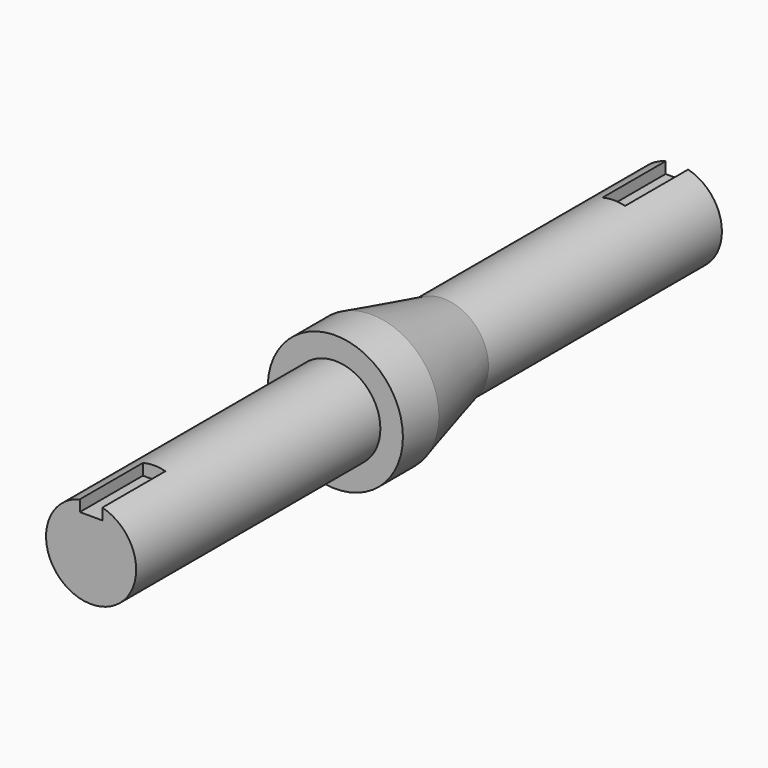
from build123d import *

# Parameters (mm, degrees)
F0_R     = 4
F1_DEPTH = 65
F3_R     = 6
F4_DEPTH = 4
F5_SIZE2 = 1.99999
F5_SIZE  = 7.99999
F7_DEPTH = 7


# Not quite as in the source:
# - a fillet or chamfer is up to 0.001 mm smaller than in the source, because OpenCascade refuses the exact size
# - a pattern or mirror of a feature is missing from the dataset's text; its kind, count and spacing are read off the source's solid


with BuildPart() as f1:
    # F0 (on Front) → F1 (new body)
    with BuildSketch(Plane.XZ):
        Circle(F0_R)
    extrude(amount=F1_DEPTH)

    # F3 (on offset) → F4 (join)
    with BuildSketch(Plane.XZ.offset(37.9)):
        Circle(F3_R)
    extrude(amount=-F4_DEPTH)

    # F5 (size 8 and 2 in the source; OpenCascade refuses exactly that, so slightly less here)
    f5_edges = [f1.edges().sort_by_distance(p)[0] for p in [
        (-4, -33.9, 0),
    ]]
    f5_side = f1.faces().sort_by_distance((-4, -16.95, 0))[0]
    chamfer(f5_edges, length=F5_SIZE, length2=F5_SIZE2, reference=f5_side)

    # F6 (on face) → F7 (cut)
    with BuildSketch(Plane.XZ.offset(65)):
        Polygon((0, 4.4108442962), (-1, 3.8729833462), (-1, 2.8729833462), (1, 2.8729833462), (1, 3.8729833462), align=None)
    f7 = extrude(amount=-F7_DEPTH, mode=Mode.SUBTRACT)

    # F7_copies: F7 across plane
    add(f7.mirror(Plane.ZX.offset(-32.5)), mode=Mode.SUBTRACT)


solid = f1.part
